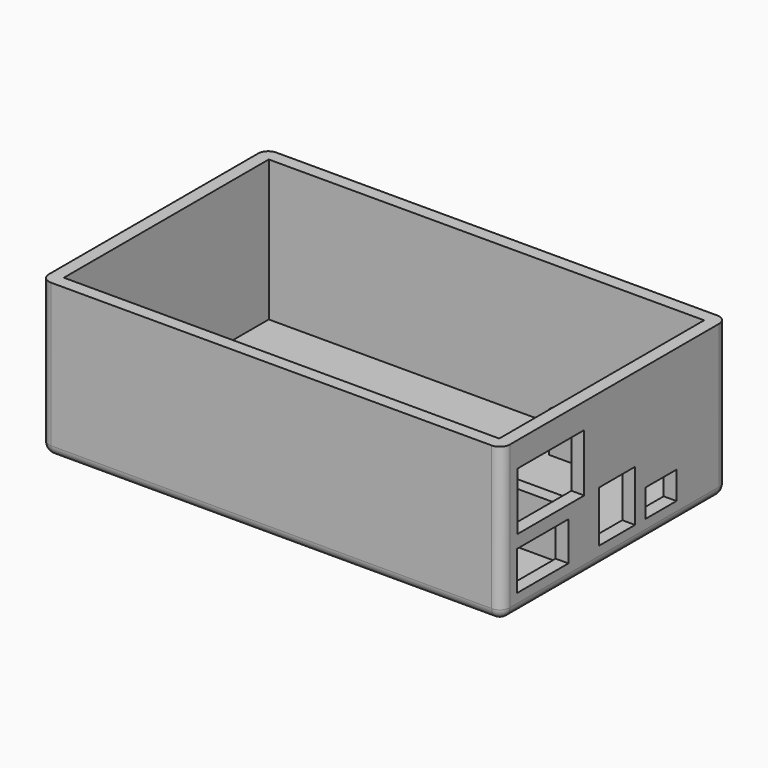
from build123d import *

# Parameters (mm, degrees)
F0_W     = 33.02
F0_H     = 41.275
F0_W_2   = 3.175
F1_DEPTH = 3.175
F0_H_2   = 19.05
F2_DEPTH = 15.875
F3_DEPTH = 38.1
F4_W     = 15.875
F4_H     = 9.652
F4_W_2   = 11.1252
F4_H_2   = 12.7
F4_W_3   = 9.652
F4_H_3   = 6.858
F4_W_4   = 20.6375
F4_H_4   = 14.2875
F5_DEPTH = 6.604
F6_W     = 3.175
F6_H     = 9.9507730049
F7_DEPTH = 7.62
F8_R     = 3
F9_R     = 2.5
F10_R    = 2.5
F11_R    = 2.5
F12_R    = 2.5
F13_R    = 2.5


# Not quite as in the source:
# - a feature names something its author has since deleted; it is built from what else it names


with BuildPart() as f1:
    # F0 (on Top) → F1 (new body)
    with BuildSketch(Plane.XY):
        with Locations((24.2028696799, 20.6375)):
            Rectangle(F0_W, F0_H)
        Polygon((4.5178696799, 0), (4.5178696799, 41.275), (-67.2371303201, 41.275), (-67.2371303201, -22.225), (4.5178696799, -22.225), align=None)
        with Locations((6.1053696799, 20.6375)):
            Rectangle(F0_W_2, F0_H)
    extrude(amount=F1_DEPTH)


with BuildPart() as f1b:
    # F0 (on Top) → F1, piece 2 (new body)
    with BuildSketch(Plane.XY):
        with Locations((24.2028696799, -12.7)):
            Rectangle(F0_W, F0_H_2)
    extrude(amount=F1_DEPTH)


with BuildPart() as f2:
    # F0 (on Top) → F2 (new body)
    with BuildSketch(Plane.XY):
        Polygon((40.7128696799, -3.175), (40.7128696799, 0), (7.6928696799, 0), (4.5178696799, 0), (4.5178696799, -22.225), (7.6928696799, -22.225), (7.6928696799, -3.175), align=None)
    extrude(amount=F2_DEPTH)


with BuildPart() as f3:
    # F0 (on Top) → F3 (new body)
    with BuildSketch(Plane.XY):
        Polygon((43.8878696799, 44.45), (-70.4121303201, 44.45), (-70.4121303201, -25.4), (43.8878696799, -25.4), (43.8878696799, 0), align=None)
        Polygon((7.6928696799, 41.275), (40.7128696799, 41.275), (40.7128696799, 0), (40.7128696799, -3.175), (40.7128696799, -22.225), (7.6928696799, -22.225), (4.5178696799, -22.225), (-67.2371303201, -22.225), (-67.2371303201, 41.275), (4.5178696799, 41.275), align=None, mode=Mode.SUBTRACT)
    extrude(amount=F3_DEPTH)

    # F4 (on face) → F5 (cut)
    with BuildSketch(Plane.YZ.offset(43.8878696799)):
        with Locations((-12.6873, 9.6012)):
            Rectangle(F4_W, F4_H)
        with Locations((10.3378, 11.1252)):
            Rectangle(F4_W_2, F4_H_2)
        with Locations((23.9014, 8.2042)):
            Rectangle(F4_W_3, F4_H_3)
        with Locations((-10.1683871388, 24.74595)):
            Rectangle(F4_W_4, F4_H_4)
    extrude(amount=-F5_DEPTH, mode=Mode.SUBTRACT)

    # F6 (on face) → F7 (join)
    with BuildSketch(Plane(origin=(40.7128696799, 0, 0), x_dir=(0, -1, 0), z_dir=(-1, 0, 0))):
        with Locations((-4.2778628612, 26.9143134976)):
            Rectangle(F6_W, F6_H)
    extrude(amount=F7_DEPTH)

    # F8
    f8_edges = [f3.edges().sort_by_distance(p)[0] for p in [
        (33.09287, 5.865363, 26.914313),
    ]]
    fillet(f8_edges, radius=F8_R)

    # F9
    f9_edges = [f3.edges().sort_by_distance(p)[0] for p in [
        (-70.41213, 44.45, 19.05),
    ]]
    fillet(f9_edges, radius=F9_R)

    # F10
    f10_edges = [f3.edges().sort_by_distance(p)[0] for p in [
        (43.88787, 44.45, 19.05),
    ]]
    fillet(f10_edges, radius=F10_R)

    # F11
    f11_edges = [f3.edges().sort_by_distance(p)[0] for p in [
        (43.88787, -25.4, 19.05),
    ]]
    fillet(f11_edges, radius=F11_R)

    # F12
    f12_edges = [f3.edges().sort_by_distance(p)[0] for p in [
        (-70.41213, -25.4, 19.05),
    ]]
    fillet(f12_edges, radius=F12_R)

    # F13
    f13_edges = [f3.edges().sort_by_distance(p)[0] for p in [
        (-13.26213, -25.4, 0),
        (-69.679897, -24.667767, 0),
        (-70.41213, 9.525, 0),
        (-69.679897, 43.717767, 0),
        (-13.26213, 44.45, 0),
        (43.155637, 43.717767, 0),
        (43.88787, 9.525, 0),
        (43.155637, -24.667767, 0),
    ]]
    fillet(f13_edges, radius=F13_R)


solid = Compound([f1.part, f1b.part, f2.part, f3.part])
